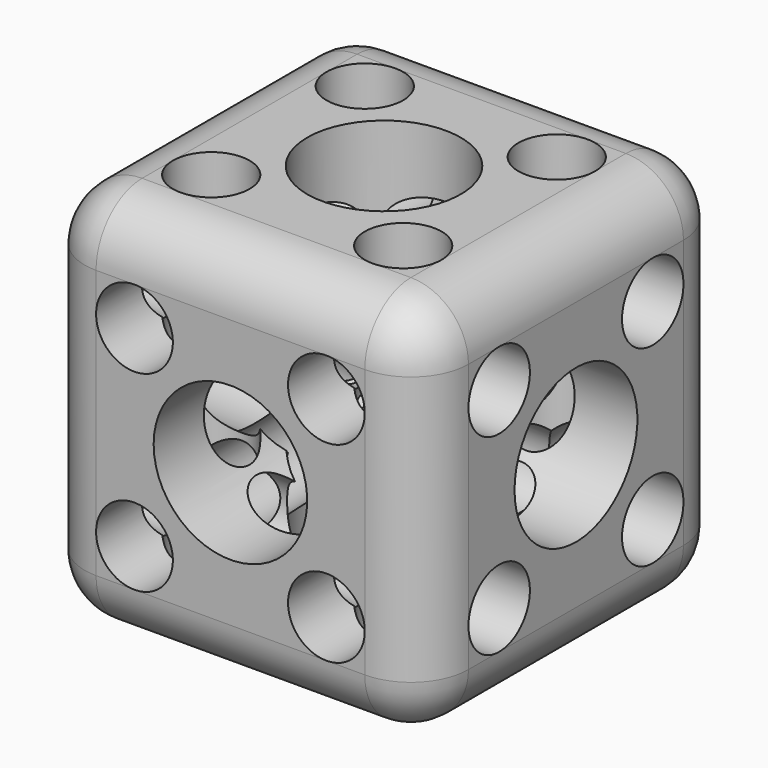
from build123d import *

# Parameters (mm, degrees)
F0_W     = 20
F0_H     = 20
F1_DEPTH = 10
F3_D     = 4
F5_D     = 4
F7_D     = 4
F8_R     = 2.99999
F10_D    = 8
F12_D    = 8
F14_D    = 8


# Not quite as in the source:
# - a fillet or chamfer is up to 0.001 mm smaller than in the source, because OpenCascade refuses the exact size


with BuildPart() as f1:
    # F0 (on Top) → F1 (new body, symmetric)
    with BuildSketch(Plane.XY):
        Rectangle(F0_W, F0_H)
    extrude(amount=F1_DEPTH, both=True)

    # F3 (through all)
    with Locations(Plane.XY.offset(10)):
        with Locations((-5, 5), (5, 5), (5, -5), (-5, -5)):
            Hole(F3_D / 2)

    # F5 (through all)
    with Locations(Plane.XZ.offset(10)):
        with Locations((-5, 5), (5, 5), (5, -5), (-5, -5)):
            Hole(F5_D / 2)

    # F7 (through all)
    with Locations(Plane.YZ.offset(10)):
        with Locations((-5, 5), (5, 5), (5, -5), (-5, -5)):
            Hole(F7_D / 2)

    # F8 (radius 3 in the source; OpenCascade refuses exactly that, so slightly less here)
    f8_edges = [f1.edges().sort_by_distance(p)[0] for p in [
        (10, 0, 10),
        (10, -10, 0),
        (10, 10, 0),
        (10, 0, -10),
        (0, 10, 10),
        (0, -10, 10),
        (-10, 0, 10),
        (0, 10, -10),
        (-10, 10, 0),
        (-10, 0, -10),
        (0, -10, -10),
        (-10, -10, 0),
    ]]
    fillet(f8_edges, radius=F8_R)

    # F10 (through all)
    with Locations(Plane.XY.offset(10)):
        with Locations((0, 0)):
            Hole(F10_D / 2)

    # F12 (through all)
    with Locations(Plane.XZ.offset(10)):
        with Locations((0, 0)):
            Hole(F12_D / 2)

    # F14 (through all)
    with Locations(Plane.YZ.offset(10)):
        with Locations((0, 0)):
            Hole(F14_D / 2)


solid = f1.part
